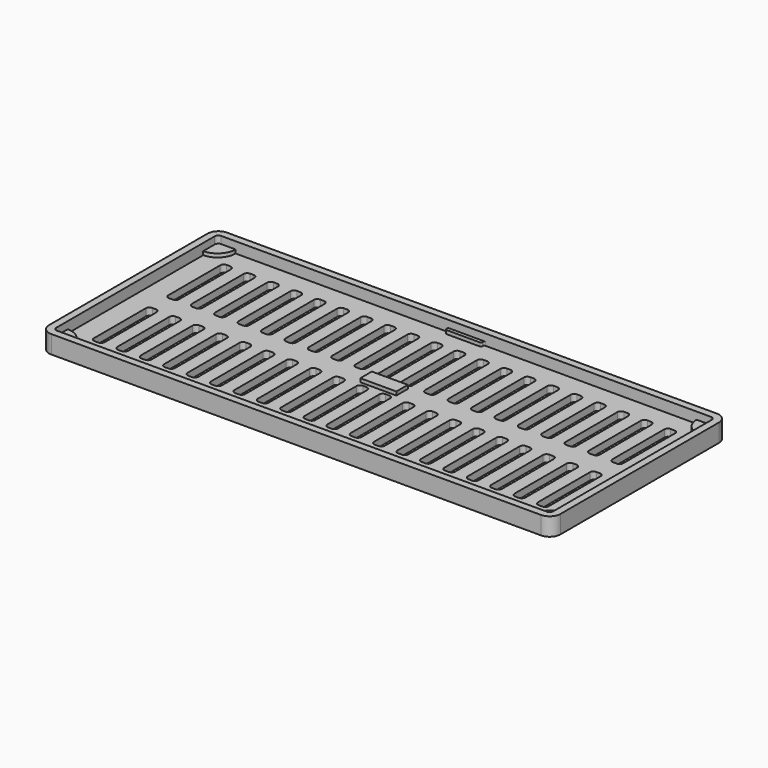
from build123d import *

# Parameters (mm, degrees)
F0_W     = 10
F0_H     = 4
F1_DEPTH = 2
F0_H_2   = 3
F2_DEPTH = 3
F3_DEPTH = 5


# Not quite as in the source:
# - a feature names something its author has since deleted; it is built from what else it names


with BuildPart() as f1:
    # F0 (on Top) → F1 (new body)
    with BuildSketch(Plane.XY):
        with BuildLine():
            ThreePointArc((0, -52), (3.5355339059, -53.4644660941), (5, -57))
            Line((5, -57), (32.5279645622, -57))
            Line((32.5279645622, -57), (32.5279645622, -54))
            Line((32.5279645622, -54), (42.5279645622, -54))
            Line((42.5279645622, -54), (42.5279645622, -57))
            Line((42.5279645622, -57), (95.4720354378, -57))
            Line((95.4720354378, -57), (95.4720354378, -54))
            Line((95.4720354378, -54), (105.4720354378, -54))
            Line((105.4720354378, -54), (105.4720354378, -57))
            Line((105.4720354378, -57), (133, -57))
            ThreePointArc((133, -57), (134.4644660941, -53.4644660941), (138, -52))
            Line((138, -52), (138, -5))
            ThreePointArc((138, -5), (134.4644660941, -3.5355339059), (133, 0))
            Line((133, 0), (74.4336718904, 0))
            ThreePointArc((74.4336718904, 0), (74.1270195559, -0.1270195559), (74, -0.4336718904))
            Line((74, -0.4336718904), (74, -0.6351635229))
            ThreePointArc((74, -0.6351635229), (73.8931418699, -0.8931418699), (73.6351635229, -1))
            Line((73.6351635229, -1), (69, -1))
            Line((69, -1), (64.3648364771, -1))
            ThreePointArc((64.3648364771, -1), (64.1068581301, -0.8931418699), (64, -0.6351635229))
            Line((64, -0.6351635229), (64, -0.3648364771))
            ThreePointArc((64, -0.3648364771), (63.8931418699, -0.1068581301), (63.6351635229, 0))
            Line((63.6351635229, 0), (5, 0))
            ThreePointArc((5, 0), (3.5355339059, -3.5355339059), (0, -5))
            Line((0, -5), (0, -52))
        make_face()
        with BuildLine():
            Line((8.84595697, -32.2402366698), (8.84595697, -50.2402366698))
            ThreePointArc((8.84595697, -50.2402366698), (8.5530637512, -50.947343451), (7.84595697, -51.2402366698))
            Line((7.84595697, -51.2402366698), (6.84595697, -51.2402366698))
            ThreePointArc((6.84595697, -51.2402366698), (6.1388501888, -50.947343451), (5.84595697, -50.2402366698))
            Line((5.84595697, -50.2402366698), (5.84595697, -32.2402366698))
            ThreePointArc((5.84595697, -32.2402366698), (6.1388501888, -31.5331298886), (6.84595697, -31.2402366698))
            Line((6.84595697, -31.2402366698), (7.84595697, -31.2402366698))
            ThreePointArc((7.84595697, -31.2402366698), (8.5530637512, -31.5331298886), (8.84595697, -32.2402366698))
        make_face(mode=Mode.SUBTRACT)
        with BuildLine():
            ThreePointArc((14.34595697, -31.2402366698), (15.0530637512, -31.5331298886), (15.34595697, -32.2402366698))
            Line((15.34595697, -32.2402366698), (15.34595697, -50.2402366698))
            ThreePointArc((15.34595697, -50.2402366698), (15.0530637512, -50.947343451), (14.34595697, -51.2402366698))
            Line((14.34595697, -51.2402366698), (13.34595697, -51.2402366698))
            ThreePointArc((13.34595697, -51.2402366698), (12.6388501888, -50.947343451), (12.34595697, -50.2402366698))
            Line((12.34595697, -50.2402366698), (12.34595697, -32.2402366698))
            ThreePointArc((12.34595697, -32.2402366698), (12.6388501888, -31.5331298886), (13.34595697, -31.2402366698))
            Line((13.34595697, -31.2402366698), (14.34595697, -31.2402366698))
        make_face(mode=Mode.SUBTRACT)
        with BuildLine():
            ThreePointArc((20.84595697, -31.2402366698), (21.5530637512, -31.5331298886), (21.84595697, -32.2402366698))
            Line((21.84595697, -32.2402366698), (21.84595697, -50.2402366698))
            ThreePointArc((21.84595697, -50.2402366698), (21.5530637512, -50.947343451), (20.84595697, -51.2402366698))
            Line((20.84595697, -51.2402366698), (19.84595697, -51.2402366698))
            ThreePointArc((19.84595697, -51.2402366698), (19.1388501888, -50.947343451), (18.84595697, -50.2402366698))
            Line((18.84595697, -50.2402366698), (18.84595697, -32.2402366698))
            ThreePointArc((18.84595697, -32.2402366698), (19.1388501888, -31.5331298886), (19.84595697, -31.2402366698))
            Line((19.84595697, -31.2402366698), (20.84595697, -31.2402366698))
        make_face(mode=Mode.SUBTRACT)
        with BuildLine():
            ThreePointArc((27.34595697, -31.2402366698), (28.0530637512, -31.5331298886), (28.34595697, -32.2402366698))
            Line((28.34595697, -32.2402366698), (28.34595697, -50.2402366698))
            ThreePointArc((28.34595697, -50.2402366698), (28.0530637512, -50.947343451), (27.34595697, -51.2402366698))
            Line((27.34595697, -51.2402366698), (26.34595697, -51.2402366698))
            ThreePointArc((26.34595697, -51.2402366698), (25.6388501888, -50.947343451), (25.34595697, -50.2402366698))
            Line((25.34595697, -50.2402366698), (25.34595697, -32.2402366698))
            ThreePointArc((25.34595697, -32.2402366698), (25.6388501888, -31.5331298886), (26.34595697, -31.2402366698))
            Line((26.34595697, -31.2402366698), (27.34595697, -31.2402366698))
        make_face(mode=Mode.SUBTRACT)
        with BuildLine():
            ThreePointArc((33.84595697, -31.2402366698), (34.5530637512, -31.5331298886), (34.84595697, -32.2402366698))
            Line((34.84595697, -32.2402366698), (34.84595697, -50.2402366698))
            ThreePointArc((34.84595697, -50.2402366698), (34.5530637512, -50.947343451), (33.84595697, -51.2402366698))
            Line((33.84595697, -51.2402366698), (32.84595697, -51.2402366698))
            ThreePointArc((32.84595697, -51.2402366698), (32.1388501888, -50.947343451), (31.84595697, -50.2402366698))
            Line((31.84595697, -50.2402366698), (31.84595697, -32.2402366698))
            ThreePointArc((31.84595697, -32.2402366698), (32.1388501888, -31.5331298886), (32.84595697, -31.2402366698))
            Line((32.84595697, -31.2402366698), (33.84595697, -31.2402366698))
        make_face(mode=Mode.SUBTRACT)
        with BuildLine():
            ThreePointArc((40.34595697, -31.2402366698), (41.0530637512, -31.5331298886), (41.34595697, -32.2402366698))
            Line((41.34595697, -32.2402366698), (41.34595697, -50.2402366698))
            ThreePointArc((41.34595697, -50.2402366698), (41.0530637512, -50.947343451), (40.34595697, -51.2402366698))
            Line((40.34595697, -51.2402366698), (39.34595697, -51.2402366698))
            ThreePointArc((39.34595697, -51.2402366698), (38.6388501888, -50.947343451), (38.34595697, -50.2402366698))
            Line((38.34595697, -50.2402366698), (38.34595697, -32.2402366698))
            ThreePointArc((38.34595697, -32.2402366698), (38.6388501888, -31.5331298886), (39.34595697, -31.2402366698))
            Line((39.34595697, -31.2402366698), (40.34595697, -31.2402366698))
        make_face(mode=Mode.SUBTRACT)
        with BuildLine():
            ThreePointArc((46.84595697, -31.2402366698), (47.5530637512, -31.5331298886), (47.84595697, -32.2402366698))
            Line((47.84595697, -32.2402366698), (47.84595697, -50.2402366698))
            ThreePointArc((47.84595697, -50.2402366698), (47.5530637512, -50.947343451), (46.84595697, -51.2402366698))
            Line((46.84595697, -51.2402366698), (45.84595697, -51.2402366698))
            ThreePointArc((45.84595697, -51.2402366698), (45.1388501888, -50.947343451), (44.84595697, -50.2402366698))
            Line((44.84595697, -50.2402366698), (44.84595697, -32.2402366698))
            ThreePointArc((44.84595697, -32.2402366698), (45.1388501888, -31.5331298886), (45.84595697, -31.2402366698))
            Line((45.84595697, -31.2402366698), (46.84595697, -31.2402366698))
        make_face(mode=Mode.SUBTRACT)
        with BuildLine():
            ThreePointArc((53.34595697, -31.2402366698), (54.0530637512, -31.5331298886), (54.34595697, -32.2402366698))
            Line((54.34595697, -32.2402366698), (54.34595697, -50.2402366698))
            ThreePointArc((54.34595697, -50.2402366698), (54.0530637512, -50.947343451), (53.34595697, -51.2402366698))
            Line((53.34595697, -51.2402366698), (52.34595697, -51.2402366698))
            ThreePointArc((52.34595697, -51.2402366698), (51.6388501888, -50.947343451), (51.34595697, -50.2402366698))
            Line((51.34595697, -50.2402366698), (51.34595697, -32.2402366698))
            ThreePointArc((51.34595697, -32.2402366698), (51.6388501888, -31.5331298886), (52.34595697, -31.2402366698))
            Line((52.34595697, -31.2402366698), (53.34595697, -31.2402366698))
        make_face(mode=Mode.SUBTRACT)
        with BuildLine():
            ThreePointArc((59.84595697, -31.2402366698), (60.5530637512, -31.5331298886), (60.84595697, -32.2402366698))
            Line((60.84595697, -32.2402366698), (60.84595697, -50.2402366698))
            ThreePointArc((60.84595697, -50.2402366698), (60.5530637512, -50.947343451), (59.84595697, -51.2402366698))
            Line((59.84595697, -51.2402366698), (58.84595697, -51.2402366698))
            ThreePointArc((58.84595697, -51.2402366698), (58.1388501888, -50.947343451), (57.84595697, -50.2402366698))
            Line((57.84595697, -50.2402366698), (57.84595697, -32.2402366698))
            ThreePointArc((57.84595697, -32.2402366698), (58.1388501888, -31.5331298886), (58.84595697, -31.2402366698))
            Line((58.84595697, -31.2402366698), (59.84595697, -31.2402366698))
        make_face(mode=Mode.SUBTRACT)
        with BuildLine():
            ThreePointArc((66.34595697, -31.2402366698), (67.0530637512, -31.5331298886), (67.34595697, -32.2402366698))
            Line((67.34595697, -32.2402366698), (67.34595697, -50.2402366698))
            ThreePointArc((67.34595697, -50.2402366698), (67.0530637512, -50.947343451), (66.34595697, -51.2402366698))
            Line((66.34595697, -51.2402366698), (65.34595697, -51.2402366698))
            ThreePointArc((65.34595697, -51.2402366698), (64.6388501888, -50.947343451), (64.34595697, -50.2402366698))
            Line((64.34595697, -50.2402366698), (64.34595697, -32.2402366698))
            ThreePointArc((64.34595697, -32.2402366698), (64.6388501888, -31.5331298886), (65.34595697, -31.2402366698))
            Line((65.34595697, -31.2402366698), (66.34595697, -31.2402366698))
        make_face(mode=Mode.SUBTRACT)
        with BuildLine():
            ThreePointArc((70.65404303, -32.2402366698), (70.9469362488, -31.5331298886), (71.65404303, -31.2402366698))
            Line((71.65404303, -31.2402366698), (72.65404303, -31.2402366698))
            ThreePointArc((72.65404303, -31.2402366698), (73.3611498112, -31.5331298886), (73.65404303, -32.2402366698))
            Line((73.65404303, -32.2402366698), (73.65404303, -50.2402366698))
            ThreePointArc((73.65404303, -50.2402366698), (73.3611498112, -50.947343451), (72.65404303, -51.2402366698))
            Line((72.65404303, -51.2402366698), (71.65404303, -51.2402366698))
            ThreePointArc((71.65404303, -51.2402366698), (70.9469362488, -50.947343451), (70.65404303, -50.2402366698))
            Line((70.65404303, -50.2402366698), (70.65404303, -32.2402366698))
        make_face(mode=Mode.SUBTRACT)
        with BuildLine():
            ThreePointArc((78.15404303, -51.2402366698), (77.4469362488, -50.947343451), (77.15404303, -50.2402366698))
            Line((77.15404303, -50.2402366698), (77.15404303, -32.2402366698))
            ThreePointArc((77.15404303, -32.2402366698), (77.4469362488, -31.5331298886), (78.15404303, -31.2402366698))
            Line((78.15404303, -31.2402366698), (79.15404303, -31.2402366698))
            ThreePointArc((79.15404303, -31.2402366698), (79.8611498112, -31.5331298886), (80.15404303, -32.2402366698))
            Line((80.15404303, -32.2402366698), (80.15404303, -50.2402366698))
            ThreePointArc((80.15404303, -50.2402366698), (79.8611498112, -50.947343451), (79.15404303, -51.2402366698))
            Line((79.15404303, -51.2402366698), (78.15404303, -51.2402366698))
        make_face(mode=Mode.SUBTRACT)
        with BuildLine():
            ThreePointArc((83.65404303, -32.2402366698), (83.9469362488, -31.5331298886), (84.65404303, -31.2402366698))
            Line((84.65404303, -31.2402366698), (85.65404303, -31.2402366698))
            ThreePointArc((85.65404303, -31.2402366698), (86.3611498112, -31.5331298886), (86.65404303, -32.2402366698))
            Line((86.65404303, -32.2402366698), (86.65404303, -50.2402366698))
            ThreePointArc((86.65404303, -50.2402366698), (86.3611498112, -50.947343451), (85.65404303, -51.2402366698))
            Line((85.65404303, -51.2402366698), (84.65404303, -51.2402366698))
            ThreePointArc((84.65404303, -51.2402366698), (83.9469362488, -50.947343451), (83.65404303, -50.2402366698))
            Line((83.65404303, -50.2402366698), (83.65404303, -32.2402366698))
        make_face(mode=Mode.SUBTRACT)
        with BuildLine():
            ThreePointArc((92.15404303, -31.2402366698), (92.8611498112, -31.5331298886), (93.15404303, -32.2402366698))
            Line((93.15404303, -32.2402366698), (93.15404303, -50.2402366698))
            ThreePointArc((93.15404303, -50.2402366698), (92.8611498112, -50.947343451), (92.15404303, -51.2402366698))
            Line((92.15404303, -51.2402366698), (91.15404303, -51.2402366698))
            ThreePointArc((91.15404303, -51.2402366698), (90.4469362488, -50.947343451), (90.15404303, -50.2402366698))
            Line((90.15404303, -50.2402366698), (90.15404303, -32.2402366698))
            ThreePointArc((90.15404303, -32.2402366698), (90.4469362488, -31.5331298886), (91.15404303, -31.2402366698))
            Line((91.15404303, -31.2402366698), (92.15404303, -31.2402366698))
        make_face(mode=Mode.SUBTRACT)
        with BuildLine():
            ThreePointArc((99.65404303, -50.2402366698), (99.3611498112, -50.947343451), (98.65404303, -51.2402366698))
            Line((98.65404303, -51.2402366698), (97.65404303, -51.2402366698))
            ThreePointArc((97.65404303, -51.2402366698), (96.9469362488, -50.947343451), (96.65404303, -50.2402366698))
            Line((96.65404303, -50.2402366698), (96.65404303, -32.2402366698))
            ThreePointArc((96.65404303, -32.2402366698), (96.9469362488, -31.5331298886), (97.65404303, -31.2402366698))
            Line((97.65404303, -31.2402366698), (98.65404303, -31.2402366698))
            ThreePointArc((98.65404303, -31.2402366698), (99.3611498112, -31.5331298886), (99.65404303, -32.2402366698))
            Line((99.65404303, -32.2402366698), (99.65404303, -50.2402366698))
        make_face(mode=Mode.SUBTRACT)
        with BuildLine():
            ThreePointArc((103.15404303, -32.2402366698), (103.4469362488, -31.5331298886), (104.15404303, -31.2402366698))
            Line((104.15404303, -31.2402366698), (105.15404303, -31.2402366698))
            ThreePointArc((105.15404303, -31.2402366698), (105.8611498112, -31.5331298886), (106.15404303, -32.2402366698))
            Line((106.15404303, -32.2402366698), (106.15404303, -50.2402366698))
            ThreePointArc((106.15404303, -50.2402366698), (105.8611498112, -50.947343451), (105.15404303, -51.2402366698))
            Line((105.15404303, -51.2402366698), (104.15404303, -51.2402366698))
            ThreePointArc((104.15404303, -51.2402366698), (103.4469362488, -50.947343451), (103.15404303, -50.2402366698))
            Line((103.15404303, -50.2402366698), (103.15404303, -32.2402366698))
        make_face(mode=Mode.SUBTRACT)
        with BuildLine():
            ThreePointArc((109.65404303, -32.2402366698), (109.9469362488, -31.5331298886), (110.65404303, -31.2402366698))
            Line((110.65404303, -31.2402366698), (111.65404303, -31.2402366698))
            ThreePointArc((111.65404303, -31.2402366698), (112.3611498112, -31.5331298886), (112.65404303, -32.2402366698))
            Line((112.65404303, -32.2402366698), (112.65404303, -50.2402366698))
            ThreePointArc((112.65404303, -50.2402366698), (112.3611498112, -50.947343451), (111.65404303, -51.2402366698))
            Line((111.65404303, -51.2402366698), (110.65404303, -51.2402366698))
            ThreePointArc((110.65404303, -51.2402366698), (109.9469362488, -50.947343451), (109.65404303, -50.2402366698))
            Line((109.65404303, -50.2402366698), (109.65404303, -32.2402366698))
        make_face(mode=Mode.SUBTRACT)
        with BuildLine():
            ThreePointArc((117.15404303, -51.2402366698), (116.4469362488, -50.947343451), (116.15404303, -50.2402366698))
            Line((116.15404303, -50.2402366698), (116.15404303, -32.2402366698))
            ThreePointArc((116.15404303, -32.2402366698), (116.4469362488, -31.5331298886), (117.15404303, -31.2402366698))
            Line((117.15404303, -31.2402366698), (118.15404303, -31.2402366698))
            ThreePointArc((118.15404303, -31.2402366698), (118.8611498112, -31.5331298886), (119.15404303, -32.2402366698))
            Line((119.15404303, -32.2402366698), (119.15404303, -50.2402366698))
            ThreePointArc((119.15404303, -50.2402366698), (118.8611498112, -50.947343451), (118.15404303, -51.2402366698))
            Line((118.15404303, -51.2402366698), (117.15404303, -51.2402366698))
        make_face(mode=Mode.SUBTRACT)
        with BuildLine():
            ThreePointArc((124.65404303, -31.2402366698), (125.3611498112, -31.5331298886), (125.65404303, -32.2402366698))
            Line((125.65404303, -32.2402366698), (125.65404303, -50.2402366698))
            ThreePointArc((125.65404303, -50.2402366698), (125.3611498112, -50.947343451), (124.65404303, -51.2402366698))
            Line((124.65404303, -51.2402366698), (123.65404303, -51.2402366698))
            ThreePointArc((123.65404303, -51.2402366698), (122.9469362488, -50.947343451), (122.65404303, -50.2402366698))
            Line((122.65404303, -50.2402366698), (122.65404303, -32.2402366698))
            ThreePointArc((122.65404303, -32.2402366698), (122.9469362488, -31.5331298886), (123.65404303, -31.2402366698))
            Line((123.65404303, -31.2402366698), (124.65404303, -31.2402366698))
        make_face(mode=Mode.SUBTRACT)
        with BuildLine():
            ThreePointArc((130.15404303, -51.2402366698), (129.4469362488, -50.947343451), (129.15404303, -50.2402366698))
            Line((129.15404303, -50.2402366698), (129.15404303, -32.2402366698))
            ThreePointArc((129.15404303, -32.2402366698), (129.4469362488, -31.5331298886), (130.15404303, -31.2402366698))
            Line((130.15404303, -31.2402366698), (131.15404303, -31.2402366698))
            ThreePointArc((131.15404303, -31.2402366698), (131.8611498112, -31.5331298886), (132.15404303, -32.2402366698))
            Line((132.15404303, -32.2402366698), (132.15404303, -50.2402366698))
            ThreePointArc((132.15404303, -50.2402366698), (131.8611498112, -50.947343451), (131.15404303, -51.2402366698))
            Line((131.15404303, -51.2402366698), (130.15404303, -51.2402366698))
        make_face(mode=Mode.SUBTRACT)
        with BuildLine():
            ThreePointArc((5.84595697, -6.4131369293), (6.1388501888, -5.7060301481), (6.84595697, -5.4131369293))
            Line((6.84595697, -5.4131369293), (7.84595697, -5.4131369293))
            ThreePointArc((7.84595697, -5.4131369293), (8.5530637512, -5.7060301481), (8.84595697, -6.4131369293))
            Line((8.84595697, -6.4131369293), (8.84595697, -24.4131369293))
            ThreePointArc((8.84595697, -24.4131369293), (8.5530637512, -25.1202437105), (7.84595697, -25.4131369293))
            Line((7.84595697, -25.4131369293), (6.84595697, -25.4131369293))
            ThreePointArc((6.84595697, -25.4131369293), (6.1388501888, -25.1202437105), (5.84595697, -24.4131369293))
            Line((5.84595697, -24.4131369293), (5.84595697, -6.4131369293))
        make_face(mode=Mode.SUBTRACT)
        with BuildLine():
            Line((15.34595697, -6.4131369293), (15.34595697, -24.4131369293))
            ThreePointArc((15.34595697, -24.4131369293), (15.0530637512, -25.1202437105), (14.34595697, -25.4131369293))
            Line((14.34595697, -25.4131369293), (13.34595697, -25.4131369293))
            ThreePointArc((13.34595697, -25.4131369293), (12.6388501888, -25.1202437105), (12.34595697, -24.4131369293))
            Line((12.34595697, -24.4131369293), (12.34595697, -6.4131369293))
            ThreePointArc((12.34595697, -6.4131369293), (12.6388501888, -5.7060301481), (13.34595697, -5.4131369293))
            Line((13.34595697, -5.4131369293), (14.34595697, -5.4131369293))
            ThreePointArc((14.34595697, -5.4131369293), (15.0530637512, -5.7060301481), (15.34595697, -6.4131369293))
        make_face(mode=Mode.SUBTRACT)
        with BuildLine():
            Line((21.84595697, -6.4131369293), (21.84595697, -24.4131369293))
            ThreePointArc((21.84595697, -24.4131369293), (21.5530637512, -25.1202437105), (20.84595697, -25.4131369293))
            Line((20.84595697, -25.4131369293), (19.84595697, -25.4131369293))
            ThreePointArc((19.84595697, -25.4131369293), (19.1388501888, -25.1202437105), (18.84595697, -24.4131369293))
            Line((18.84595697, -24.4131369293), (18.84595697, -6.4131369293))
            ThreePointArc((18.84595697, -6.4131369293), (19.1388501888, -5.7060301481), (19.84595697, -5.4131369293))
            Line((19.84595697, -5.4131369293), (20.84595697, -5.4131369293))
            ThreePointArc((20.84595697, -5.4131369293), (21.5530637512, -5.7060301481), (21.84595697, -6.4131369293))
        make_face(mode=Mode.SUBTRACT)
        with BuildLine():
            Line((28.34595697, -6.4131369293), (28.34595697, -24.4131369293))
            ThreePointArc((28.34595697, -24.4131369293), (28.0530637512, -25.1202437105), (27.34595697, -25.4131369293))
            Line((27.34595697, -25.4131369293), (26.34595697, -25.4131369293))
            ThreePointArc((26.34595697, -25.4131369293), (25.6388501888, -25.1202437105), (25.34595697, -24.4131369293))
            Line((25.34595697, -24.4131369293), (25.34595697, -6.4131369293))
            ThreePointArc((25.34595697, -6.4131369293), (25.6388501888, -5.7060301481), (26.34595697, -5.4131369293))
            Line((26.34595697, -5.4131369293), (27.34595697, -5.4131369293))
            ThreePointArc((27.34595697, -5.4131369293), (28.0530637512, -5.7060301481), (28.34595697, -6.4131369293))
        make_face(mode=Mode.SUBTRACT)
        with Locations((68.8843362331, -28.3266867995)):
            Rectangle(F0_W, F0_H, mode=Mode.SUBTRACT)
        with BuildLine():
            Line((34.84595697, -6.4131369293), (34.84595697, -24.4131369293))
            ThreePointArc((34.84595697, -24.4131369293), (34.5530637512, -25.1202437105), (33.84595697, -25.4131369293))
            Line((33.84595697, -25.4131369293), (32.84595697, -25.4131369293))
            ThreePointArc((32.84595697, -25.4131369293), (32.1388501888, -25.1202437105), (31.84595697, -24.4131369293))
            Line((31.84595697, -24.4131369293), (31.84595697, -6.4131369293))
            ThreePointArc((31.84595697, -6.4131369293), (32.1388501888, -5.7060301481), (32.84595697, -5.4131369293))
            Line((32.84595697, -5.4131369293), (33.84595697, -5.4131369293))
            ThreePointArc((33.84595697, -5.4131369293), (34.5530637512, -5.7060301481), (34.84595697, -6.4131369293))
        make_face(mode=Mode.SUBTRACT)
        with BuildLine():
            Line((41.34595697, -6.4131369293), (41.34595697, -24.4131369293))
            ThreePointArc((41.34595697, -24.4131369293), (41.0530637512, -25.1202437105), (40.34595697, -25.4131369293))
            Line((40.34595697, -25.4131369293), (39.34595697, -25.4131369293))
            ThreePointArc((39.34595697, -25.4131369293), (38.6388501888, -25.1202437105), (38.34595697, -24.4131369293))
            Line((38.34595697, -24.4131369293), (38.34595697, -6.4131369293))
            ThreePointArc((38.34595697, -6.4131369293), (38.6388501888, -5.7060301481), (39.34595697, -5.4131369293))
            Line((39.34595697, -5.4131369293), (40.34595697, -5.4131369293))
            ThreePointArc((40.34595697, -5.4131369293), (41.0530637512, -5.7060301481), (41.34595697, -6.4131369293))
        make_face(mode=Mode.SUBTRACT)
        with BuildLine():
            Line((47.84595697, -6.4131369293), (47.84595697, -24.4131369293))
            ThreePointArc((47.84595697, -24.4131369293), (47.5530637512, -25.1202437105), (46.84595697, -25.4131369293))
            Line((46.84595697, -25.4131369293), (45.84595697, -25.4131369293))
            ThreePointArc((45.84595697, -25.4131369293), (45.1388501888, -25.1202437105), (44.84595697, -24.4131369293))
            Line((44.84595697, -24.4131369293), (44.84595697, -6.4131369293))
            ThreePointArc((44.84595697, -6.4131369293), (45.1388501888, -5.7060301481), (45.84595697, -5.4131369293))
            Line((45.84595697, -5.4131369293), (46.84595697, -5.4131369293))
            ThreePointArc((46.84595697, -5.4131369293), (47.5530637512, -5.7060301481), (47.84595697, -6.4131369293))
        make_face(mode=Mode.SUBTRACT)
        with BuildLine():
            Line((54.34595697, -6.4131369293), (54.34595697, -24.4131369293))
            ThreePointArc((54.34595697, -24.4131369293), (54.0530637512, -25.1202437105), (53.34595697, -25.4131369293))
            Line((53.34595697, -25.4131369293), (52.34595697, -25.4131369293))
            ThreePointArc((52.34595697, -25.4131369293), (51.6388501888, -25.1202437105), (51.34595697, -24.4131369293))
            Line((51.34595697, -24.4131369293), (51.34595697, -6.4131369293))
            ThreePointArc((51.34595697, -6.4131369293), (51.6388501888, -5.7060301481), (52.34595697, -5.4131369293))
            Line((52.34595697, -5.4131369293), (53.34595697, -5.4131369293))
            ThreePointArc((53.34595697, -5.4131369293), (54.0530637512, -5.7060301481), (54.34595697, -6.4131369293))
        make_face(mode=Mode.SUBTRACT)
        with BuildLine():
            Line((60.84595697, -6.4131369293), (60.84595697, -24.4131369293))
            ThreePointArc((60.84595697, -24.4131369293), (60.5530637512, -25.1202437105), (59.84595697, -25.4131369293))
            Line((59.84595697, -25.4131369293), (58.84595697, -25.4131369293))
            ThreePointArc((58.84595697, -25.4131369293), (58.1388501888, -25.1202437105), (57.84595697, -24.4131369293))
            Line((57.84595697, -24.4131369293), (57.84595697, -6.4131369293))
            ThreePointArc((57.84595697, -6.4131369293), (58.1388501888, -5.7060301481), (58.84595697, -5.4131369293))
            Line((58.84595697, -5.4131369293), (59.84595697, -5.4131369293))
            ThreePointArc((59.84595697, -5.4131369293), (60.5530637512, -5.7060301481), (60.84595697, -6.4131369293))
        make_face(mode=Mode.SUBTRACT)
        with BuildLine():
            Line((67.34595697, -6.4131369293), (67.34595697, -24.4131369293))
            ThreePointArc((67.34595697, -24.4131369293), (67.0530637512, -25.1202437105), (66.34595697, -25.4131369293))
            Line((66.34595697, -25.4131369293), (65.34595697, -25.4131369293))
            ThreePointArc((65.34595697, -25.4131369293), (64.6388501888, -25.1202437105), (64.34595697, -24.4131369293))
            Line((64.34595697, -24.4131369293), (64.34595697, -6.4131369293))
            ThreePointArc((64.34595697, -6.4131369293), (64.6388501888, -5.7060301481), (65.34595697, -5.4131369293))
            Line((65.34595697, -5.4131369293), (66.34595697, -5.4131369293))
            ThreePointArc((66.34595697, -5.4131369293), (67.0530637512, -5.7060301481), (67.34595697, -6.4131369293))
        make_face(mode=Mode.SUBTRACT)
        with BuildLine():
            Line((70.65404303, -24.4131369293), (70.65404303, -6.4131369293))
            ThreePointArc((70.65404303, -6.4131369293), (70.9469362488, -5.7060301481), (71.65404303, -5.4131369293))
            Line((71.65404303, -5.4131369293), (72.65404303, -5.4131369293))
            ThreePointArc((72.65404303, -5.4131369293), (73.3611498112, -5.7060301481), (73.65404303, -6.4131369293))
            Line((73.65404303, -6.4131369293), (73.65404303, -24.4131369293))
            ThreePointArc((73.65404303, -24.4131369293), (73.3611498112, -25.1202437105), (72.65404303, -25.4131369293))
            Line((72.65404303, -25.4131369293), (71.65404303, -25.4131369293))
            ThreePointArc((71.65404303, -25.4131369293), (70.9469362488, -25.1202437105), (70.65404303, -24.4131369293))
        make_face(mode=Mode.SUBTRACT)
        with BuildLine():
            Line((77.15404303, -24.4131369293), (77.15404303, -6.4131369293))
            ThreePointArc((77.15404303, -6.4131369293), (77.4469362488, -5.7060301481), (78.15404303, -5.4131369293))
            Line((78.15404303, -5.4131369293), (79.15404303, -5.4131369293))
            ThreePointArc((79.15404303, -5.4131369293), (79.8611498112, -5.7060301481), (80.15404303, -6.4131369293))
            Line((80.15404303, -6.4131369293), (80.15404303, -24.4131369293))
            ThreePointArc((80.15404303, -24.4131369293), (79.8611498112, -25.1202437105), (79.15404303, -25.4131369293))
            Line((79.15404303, -25.4131369293), (78.15404303, -25.4131369293))
            ThreePointArc((78.15404303, -25.4131369293), (77.4469362488, -25.1202437105), (77.15404303, -24.4131369293))
        make_face(mode=Mode.SUBTRACT)
        with BuildLine():
            Line((83.65404303, -24.4131369293), (83.65404303, -6.4131369293))
            ThreePointArc((83.65404303, -6.4131369293), (83.9469362488, -5.7060301481), (84.65404303, -5.4131369293))
            Line((84.65404303, -5.4131369293), (85.65404303, -5.4131369293))
            ThreePointArc((85.65404303, -5.4131369293), (86.3611498112, -5.7060301481), (86.65404303, -6.4131369293))
            Line((86.65404303, -6.4131369293), (86.65404303, -24.4131369293))
            ThreePointArc((86.65404303, -24.4131369293), (86.3611498112, -25.1202437105), (85.65404303, -25.4131369293))
            Line((85.65404303, -25.4131369293), (84.65404303, -25.4131369293))
            ThreePointArc((84.65404303, -25.4131369293), (83.9469362488, -25.1202437105), (83.65404303, -24.4131369293))
        make_face(mode=Mode.SUBTRACT)
        with BuildLine():
            Line((91.15404303, -5.4131369293), (92.15404303, -5.4131369293))
            ThreePointArc((92.15404303, -5.4131369293), (92.8611498112, -5.7060301481), (93.15404303, -6.4131369293))
            Line((93.15404303, -6.4131369293), (93.15404303, -24.4131369293))
            ThreePointArc((93.15404303, -24.4131369293), (92.8611498112, -25.1202437105), (92.15404303, -25.4131369293))
            Line((92.15404303, -25.4131369293), (91.15404303, -25.4131369293))
            ThreePointArc((91.15404303, -25.4131369293), (90.4469362488, -25.1202437105), (90.15404303, -24.4131369293))
            Line((90.15404303, -24.4131369293), (90.15404303, -6.4131369293))
            ThreePointArc((90.15404303, -6.4131369293), (90.4469362488, -5.7060301481), (91.15404303, -5.4131369293))
        make_face(mode=Mode.SUBTRACT)
        with BuildLine():
            Line((97.65404303, -5.4131369293), (98.65404303, -5.4131369293))
            ThreePointArc((98.65404303, -5.4131369293), (99.3611498112, -5.7060301481), (99.65404303, -6.4131369293))
            Line((99.65404303, -6.4131369293), (99.65404303, -24.4131369293))
            ThreePointArc((99.65404303, -24.4131369293), (99.3611498112, -25.1202437105), (98.65404303, -25.4131369293))
            Line((98.65404303, -25.4131369293), (97.65404303, -25.4131369293))
            ThreePointArc((97.65404303, -25.4131369293), (96.9469362488, -25.1202437105), (96.65404303, -24.4131369293))
            Line((96.65404303, -24.4131369293), (96.65404303, -6.4131369293))
            ThreePointArc((96.65404303, -6.4131369293), (96.9469362488, -5.7060301481), (97.65404303, -5.4131369293))
        make_face(mode=Mode.SUBTRACT)
        with BuildLine():
            Line((104.15404303, -5.4131369293), (105.15404303, -5.4131369293))
            ThreePointArc((105.15404303, -5.4131369293), (105.8611498112, -5.7060301481), (106.15404303, -6.4131369293))
            Line((106.15404303, -6.4131369293), (106.15404303, -24.4131369293))
            ThreePointArc((106.15404303, -24.4131369293), (105.8611498112, -25.1202437105), (105.15404303, -25.4131369293))
            Line((105.15404303, -25.4131369293), (104.15404303, -25.4131369293))
            ThreePointArc((104.15404303, -25.4131369293), (103.4469362488, -25.1202437105), (103.15404303, -24.4131369293))
            Line((103.15404303, -24.4131369293), (103.15404303, -6.4131369293))
            ThreePointArc((103.15404303, -6.4131369293), (103.4469362488, -5.7060301481), (104.15404303, -5.4131369293))
        make_face(mode=Mode.SUBTRACT)
        with BuildLine():
            Line((109.65404303, -24.4131369293), (109.65404303, -6.4131369293))
            ThreePointArc((109.65404303, -6.4131369293), (109.9469362488, -5.7060301481), (110.65404303, -5.4131369293))
            Line((110.65404303, -5.4131369293), (111.65404303, -5.4131369293))
            ThreePointArc((111.65404303, -5.4131369293), (112.3611498112, -5.7060301481), (112.65404303, -6.4131369293))
            Line((112.65404303, -6.4131369293), (112.65404303, -24.4131369293))
            ThreePointArc((112.65404303, -24.4131369293), (112.3611498112, -25.1202437105), (111.65404303, -25.4131369293))
            Line((111.65404303, -25.4131369293), (110.65404303, -25.4131369293))
            ThreePointArc((110.65404303, -25.4131369293), (109.9469362488, -25.1202437105), (109.65404303, -24.4131369293))
        make_face(mode=Mode.SUBTRACT)
        with BuildLine():
            Line((117.15404303, -5.4131369293), (118.15404303, -5.4131369293))
            ThreePointArc((118.15404303, -5.4131369293), (118.8611498112, -5.7060301481), (119.15404303, -6.4131369293))
            Line((119.15404303, -6.4131369293), (119.15404303, -24.4131369293))
            ThreePointArc((119.15404303, -24.4131369293), (118.8611498112, -25.1202437105), (118.15404303, -25.4131369293))
            Line((118.15404303, -25.4131369293), (117.15404303, -25.4131369293))
            ThreePointArc((117.15404303, -25.4131369293), (116.4469362488, -25.1202437105), (116.15404303, -24.4131369293))
            Line((116.15404303, -24.4131369293), (116.15404303, -6.4131369293))
            ThreePointArc((116.15404303, -6.4131369293), (116.4469362488, -5.7060301481), (117.15404303, -5.4131369293))
        make_face(mode=Mode.SUBTRACT)
        with BuildLine():
            ThreePointArc((125.65404303, -24.4131369293), (125.3611498112, -25.1202437105), (124.65404303, -25.4131369293))
            Line((124.65404303, -25.4131369293), (123.65404303, -25.4131369293))
            ThreePointArc((123.65404303, -25.4131369293), (122.9469362488, -25.1202437105), (122.65404303, -24.4131369293))
            Line((122.65404303, -24.4131369293), (122.65404303, -6.4131369293))
            ThreePointArc((122.65404303, -6.4131369293), (122.9469362488, -5.7060301481), (123.65404303, -5.4131369293))
            Line((123.65404303, -5.4131369293), (124.65404303, -5.4131369293))
            ThreePointArc((124.65404303, -5.4131369293), (125.3611498112, -5.7060301481), (125.65404303, -6.4131369293))
            Line((125.65404303, -6.4131369293), (125.65404303, -24.4131369293))
        make_face(mode=Mode.SUBTRACT)
        with BuildLine():
            Line((130.15404303, -5.4131369293), (131.15404303, -5.4131369293))
            ThreePointArc((131.15404303, -5.4131369293), (131.8611498112, -5.7060301481), (132.15404303, -6.4131369293))
            Line((132.15404303, -6.4131369293), (132.15404303, -24.4131369293))
            ThreePointArc((132.15404303, -24.4131369293), (131.8611498112, -25.1202437105), (131.15404303, -25.4131369293))
            Line((131.15404303, -25.4131369293), (130.15404303, -25.4131369293))
            ThreePointArc((130.15404303, -25.4131369293), (129.4469362488, -25.1202437105), (129.15404303, -24.4131369293))
            Line((129.15404303, -24.4131369293), (129.15404303, -6.4131369293))
            ThreePointArc((129.15404303, -6.4131369293), (129.4469362488, -5.7060301481), (130.15404303, -5.4131369293))
        make_face(mode=Mode.SUBTRACT)
    extrude(amount=F1_DEPTH)

    # F0 (on Top) → F2 (join)
    with BuildSketch(Plane.XY):
        with BuildLine():
            Line((0, -1), (0, -5))
            ThreePointArc((0, -5), (3.5355339059, -3.5355339059), (5, 0))
            Line((5, 0), (1, 0))
            ThreePointArc((1, 0), (0.2928932188, -0.2928932188), (0, -1))
        make_face()
        with BuildLine():
            ThreePointArc((0, -56), (0.2928932188, -56.7071067812), (1, -57))
            Line((1, -57), (5, -57))
            ThreePointArc((5, -57), (3.5355339059, -53.4644660941), (0, -52))
            Line((0, -52), (0, -56))
        make_face()
        with Locations((37.5279645622, -55.5)):
            Rectangle(F0_W, F0_H_2)
        with Locations((68.8843362331, -28.3266867995)):
            Rectangle(F0_W, F0_H)
        with Locations((100.4720354378, -55.5)):
            Rectangle(F0_W, F0_H_2)
        with BuildLine():
            ThreePointArc((138, -52), (134.4644660941, -53.4644660941), (133, -57))
            Line((133, -57), (137, -57))
            ThreePointArc((137, -57), (137.7071067812, -56.7071067812), (138, -56))
            Line((138, -56), (138, -52))
        make_face()
        with BuildLine():
            ThreePointArc((133, 0), (134.4644660941, -3.5355339059), (138, -5))
            Line((138, -5), (138, -1))
            ThreePointArc((138, -1), (137.7071067812, -0.2928932188), (137, 0))
            Line((137, 0), (133, 0))
        make_face()
        with BuildLine():
            Line((74.4336718904, 0), (63.6351635229, 0))
            ThreePointArc((63.6351635229, 0), (63.8931418699, -0.1068581301), (64, -0.3648364771))
            Line((64, -0.3648364771), (64, -0.6351635229))
            ThreePointArc((64, -0.6351635229), (64.1068581301, -0.8931418699), (64.3648364771, -1))
            Line((64.3648364771, -1), (69, -1))
            Line((69, -1), (73.6351635229, -1))
            ThreePointArc((73.6351635229, -1), (73.8931418699, -0.8931418699), (74, -0.6351635229))
            Line((74, -0.6351635229), (74, -0.4336718904))
            ThreePointArc((74, -0.4336718904), (74.1270195559, -0.1270195559), (74.4336718904, 0))
        make_face()
    extrude(amount=F2_DEPTH)

    # F0 (on Top) → F3 (join)
    with BuildSketch(Plane.XY):
        with BuildLine():
            Line((138, -5), (138, -52))
            ThreePointArc((138, -52), (139.0215482184, -52.1054684353), (140, -52.417424305))
            Line((140, -52.417424305), (140, -4.582575695))
            ThreePointArc((140, -4.582575695), (139.0215482184, -4.8945315647), (138, -5))
        make_face()
        with BuildLine():
            Line((137, 2), (133.417424305, 2))
            ThreePointArc((133.417424305, 2), (133.1054684353, 1.0215482184), (133, 0))
            Line((133, 0), (137, 0))
            ThreePointArc((137, 0), (137.7071067812, -0.2928932188), (138, -1))
            Line((138, -1), (138, -5))
            ThreePointArc((138, -5), (139.0215482184, -4.8945315647), (140, -4.582575695))
            Line((140, -4.582575695), (140, -1))
            ThreePointArc((140, -1), (139.1213203436, 1.1213203436), (137, 2))
        make_face()
        with BuildLine():
            ThreePointArc((133, -57), (133.1054684353, -58.0215482184), (133.417424305, -59))
            Line((133.417424305, -59), (137, -59))
            ThreePointArc((137, -59), (139.1213203436, -58.1213203436), (140, -56))
            Line((140, -56), (140, -52.417424305))
            ThreePointArc((140, -52.417424305), (139.0215482184, -52.1054684353), (138, -52))
            Line((138, -52), (138, -56))
            ThreePointArc((138, -56), (137.7071067812, -56.7071067812), (137, -57))
            Line((137, -57), (133, -57))
        make_face()
        with BuildLine():
            Line((32.5279645622, -57), (5, -57))
            ThreePointArc((5, -57), (4.8945315647, -58.0215482184), (4.582575695, -59))
            Line((4.582575695, -59), (133.417424305, -59))
            ThreePointArc((133.417424305, -59), (133.1054684353, -58.0215482184), (133, -57))
            Line((133, -57), (105.4720354378, -57))
            Line((105.4720354378, -57), (95.4720354378, -57))
            Line((95.4720354378, -57), (42.5279645622, -57))
            Line((42.5279645622, -57), (32.5279645622, -57))
        make_face()
        with BuildLine():
            Line((5, -57), (1, -57))
            ThreePointArc((1, -57), (0.2928932188, -56.7071067812), (0, -56))
            Line((0, -56), (0, -52))
            ThreePointArc((0, -52), (-1.0215482184, -52.1054684353), (-2, -52.417424305))
            Line((-2, -52.417424305), (-2, -56))
            ThreePointArc((-2, -56), (-1.1213203436, -58.1213203436), (1, -59))
            Line((1, -59), (4.582575695, -59))
            ThreePointArc((4.582575695, -59), (4.8945315647, -58.0215482184), (5, -57))
        make_face()
        with BuildLine():
            ThreePointArc((-2, -52.417424305), (-1.0215482184, -52.1054684353), (0, -52))
            Line((0, -52), (0, -5))
            ThreePointArc((0, -5), (-1.0215482184, -4.8945315647), (-2, -4.582575695))
            Line((-2, -4.582575695), (-2, -52.417424305))
        make_face()
        with BuildLine():
            ThreePointArc((-2, -4.582575695), (-1.0215482184, -4.8945315647), (0, -5))
            Line((0, -5), (0, -1))
            ThreePointArc((0, -1), (0.2928932188, -0.2928932188), (1, 0))
            Line((1, 0), (5, 0))
            ThreePointArc((5, 0), (4.8945315647, 1.0215482184), (4.582575695, 2))
            Line((4.582575695, 2), (1, 2))
            ThreePointArc((1, 2), (-1.1213203436, 1.1213203436), (-2, -1))
            Line((-2, -1), (-2, -4.582575695))
        make_face()
        with BuildLine():
            ThreePointArc((4.582575695, 2), (4.8945315647, 1.0215482184), (5, 0))
            Line((5, 0), (63.6351635229, 0))
            Line((63.6351635229, 0), (74.4336718904, 0))
            Line((74.4336718904, 0), (133, 0))
            ThreePointArc((133, 0), (133.1054684353, 1.0215482184), (133.417424305, 2))
            Line((133.417424305, 2), (4.582575695, 2))
        make_face()
    extrude(amount=F3_DEPTH)


solid = f1.part
